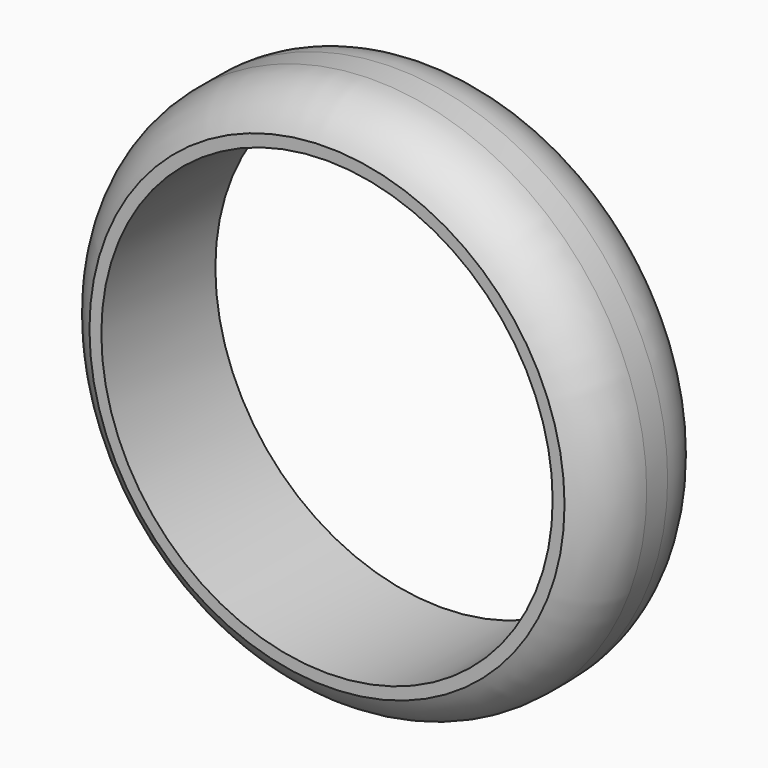
from build123d import *

# Parameters (mm, degrees)
F0_R     = 11.5
F0_R_2   = 10
F1_DEPTH = 6
F0_R_3   = 9.5
F3_DEPTH = 6


# Not quite as in the source:
# - a fillet or chamfer that OpenCascade refuses, or shapes differently, is made with other operations: its cross-section is extruded or revolved along the edge and cut away or added


with BuildPart() as f1:
    # F0 (on Front) → F1 (new body)
    with BuildSketch(Plane.XZ):
        Circle(F0_R)
        Circle(F0_R_2, mode=Mode.SUBTRACT)
    extrude(amount=F1_DEPTH)

    # F2: fillet of radius 2.75 on 3 edges, made by hand

    # F2_s1 → F2_t2 (revolve, cut)
    with BuildSketch(Plane.XY):
        with BuildLine():
            ThreePointArc((11.5, -2.4494897428), (11.0952078799, -1.0133490811), (10, 0))
            Line((10, 0), (11.5, 0))
            Line((11.5, 0), (11.5, -2.4494897428))
        make_face()
    revolve(axis=Axis((0, 0, 0), (0, -1, 0)), mode=Mode.SUBTRACT)

    # F2_s3 → F2_t4 (revolve, cut)
    with BuildSketch(Plane.XY):
        with BuildLine():
            ThreePointArc((11.5, -3.5505102572), (11.0952078799, -4.9866509189), (10, -6))
            Line((10, -6), (11.5, -6))
            Line((11.5, -6), (11.5, -3.5505102572))
        make_face()
    revolve(axis=Axis((0, -6, 0), (0, -1, 0)), mode=Mode.SUBTRACT)

    # F0 (on Front) → F3 (join)
    with BuildSketch(Plane.XZ):
        Circle(F0_R_2)
        Circle(F0_R_3, mode=Mode.SUBTRACT)
    extrude(amount=F3_DEPTH)


solid = f1.part
